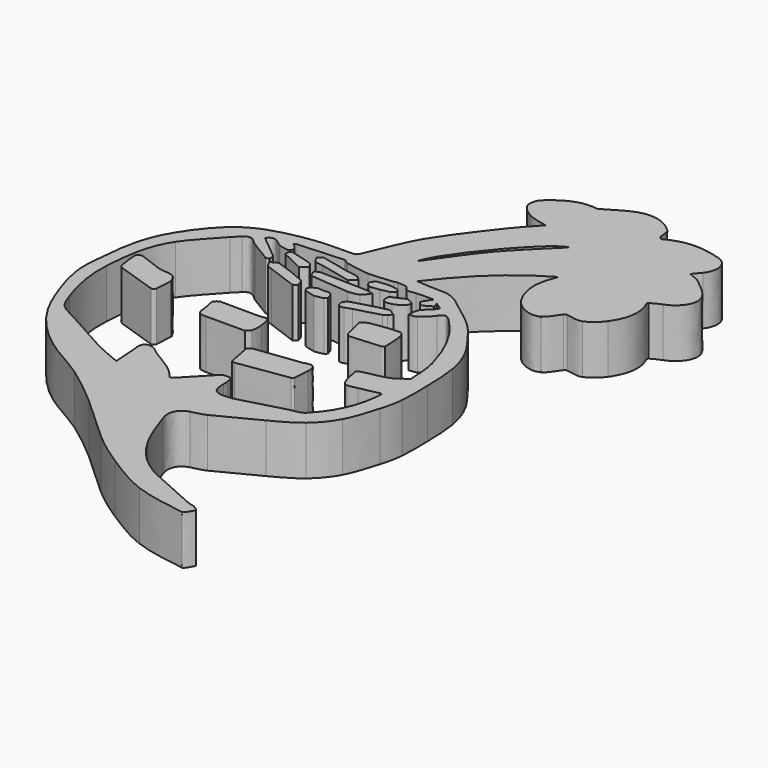
from build123d import *

# Parameters (mm, degrees)
F1_DEPTH = 6.35


# Not quite as in the source:
# - the dataset's text gives a spline's control points without its knots; the knots are read off the source's solid


with BuildPart() as f1:
    # F0 (on Top) → F1 (new body)
    with BuildSketch(Plane.XY):
        with BuildLine():
            add(Edge.make_bspline(
                [(4.2072051852, 31.8483006501), (3.3828085836, 32.0647178316), (2.4756531936, 32.1572918229), (1.7198021082, 32.5450191599)],
                knots=[0, 0, 0, 0, 1, 1, 1, 1], degree=3))
            add(Edge.make_bspline(
                [(1.435188038, 28.715078668), (2.2810654528, 29.8213807729), (3.2804193892, 30.8100077115), (4.2072051852, 31.8483006501)],
                knots=[65, 65, 65, 65, 66, 66, 66, 66], degree=3))
            add(Edge.make_bspline(
                [(-3.5365341043, 21.8426665957), (-2.081577752, 24.2562142926), (-0.2830892938, 26.4680944301), (1.435188038, 28.715078668)],
                knots=[64, 64, 64, 64, 65, 65, 65, 65], degree=3))
            add(Edge.make_bspline(
                [(-6.4304099471, 15.4801891832), (-5.4692441229, 17.6051270032), (-4.731038949, 19.8608537444), (-3.5365341043, 21.8426665957)],
                knots=[63, 63, 63, 63, 64, 64, 64, 64], degree=3))
            add(Edge.make_bspline(
                [(-6.9774600195, 14.832734411), (-6.7812364115, 14.8431127814), (-6.5458860788, 15.2246720946), (-6.4304099471, 15.4801891832)],
                knots=[62, 62, 62, 62, 63, 63, 63, 63], degree=3))
            add(Edge.make_bspline(
                [(-11.8025977362, 14.6692549639), (-10.2139829908, 14.8723974855), (-8.5851956385, 14.7481788505), (-6.9774600195, 14.832734411)],
                knots=[61, 61, 61, 61, 62, 62, 62, 62], degree=3))
            add(Edge.make_bspline(
                [(-17.1400568699, 13.4998244767), (-15.4285107292, 14.0925447424), (-13.6058328909, 14.4388122327), (-11.8025977362, 14.6692549639)],
                knots=[60, 60, 60, 60, 61, 61, 61, 61], degree=3))
            add(Edge.make_bspline(
                [(-20.7615986113, 11.3783461135), (-19.7644168919, 12.3189697367), (-18.4447816174, 13.04808378), (-17.1400568699, 13.4998244767)],
                knots=[59, 59, 59, 59, 60, 60, 60, 60], degree=3))
            add(Edge.make_bspline(
                [(-24.1170571712, 7.1628236841), (-23.1797052822, 8.6861646476), (-22.0579563004, 10.1554683595), (-20.7615986113, 11.3783461135)],
                knots=[58, 58, 58, 58, 59, 59, 59, 59], degree=3))
            add(Edge.make_bspline(
                [(-26.6270137612, -2.7980519719), (-26.4535045711, -0.8760957685), (-26.3074564955, 1.0700766324), (-25.8659064468, 2.9391487364), (-25.5188880666, 4.4080770033), (-24.908173262, 5.8770320878), (-24.1170571712, 7.1628236841)],
                knots=[56, 56, 56, 56, 57, 57, 57, 58, 58, 58, 58], degree=3))
            add(Edge.make_bspline(
                [(-26.5517102363, -5.9227191732), (-26.7292152331, -4.9059070478), (-26.7203118249, -3.8317859364), (-26.6270137612, -2.7980519719)],
                knots=[55, 55, 55, 55, 56, 56, 56, 56], degree=3))
            add(Edge.make_bspline(
                [(-25.4965222761, -9.7386877505), (-25.9495502125, -8.5018112643), (-26.3254778518, -7.2178164401), (-26.5517102363, -5.9227191732)],
                knots=[54, 54, 54, 54, 55, 55, 55, 55], degree=3))
            add(Edge.make_bspline(
                [(-23.6601943331, -13.9141716604), (-24.4193171529, -12.606201996), (-24.9740102113, -11.165083471), (-25.4965222761, -9.7386877505)],
                knots=[53, 53, 53, 53, 54, 54, 54, 54], degree=3))
            add(Edge.make_bspline(
                [(-12.9440039416, -22.9917594966), (-14.5380894559, -21.8721827318), (-16.3289349281, -21.0344846528), (-17.9390036691, -19.9351014615), (-20.2652872386, -18.3466744386), (-22.2420047659, -16.3577549513), (-23.6601943331, -13.9141716604)],
                knots=[51, 51, 51, 51, 52, 52, 52, 53, 53, 53, 53], degree=3))
            add(Edge.make_bspline(
                [(-7.8668085931, -27.0197471862), (-9.4963468352, -25.6031934862), (-11.1786082718, -24.2315322721), (-12.9440039416, -22.9917594966)],
                knots=[50, 50, 50, 50, 51, 51, 51, 51], degree=3))
            add(Edge.make_bspline(
                [(-1.9632053308, -32.4090445369), (-3.985190789, -30.6758566781), (-5.85643511, -28.7673360396), (-7.8668085931, -27.0197471862)],
                knots=[49, 49, 49, 49, 50, 50, 50, 50], degree=3))
            add(Edge.make_bspline(
                [(2.4047209204, -35.6275461519), (0.8784836675, -34.6634840383), (-0.5928313565, -33.5835435306), (-1.9632053308, -32.4090445369)],
                knots=[48, 48, 48, 48, 49, 49, 49, 49], degree=3))
            add(Edge.make_bspline(
                [(8.0590019353, -38.7449458122), (6.0608035948, -38.0082156004), (4.2254142641, -36.7776948605), (2.4047209204, -35.6275461519)],
                knots=[47, 47, 47, 47, 48, 48, 48, 48], degree=3))
            add(Edge.make_bspline(
                [(14.710813297, -40.1737014722), (12.4718206725, -39.8001605899), (10.1690292283, -39.5226263382), (8.0590019353, -38.7449458122)],
                knots=[46, 46, 46, 46, 47, 47, 47, 47], degree=3))
            add(Edge.make_bspline(
                [(15.5905075725, -38.994294877), (15.3333277993, -39.4305886967), (14.9437768726, -40.2124527519), (14.710813297, -40.1737014722)],
                knots=[45, 45, 45, 45, 46, 46, 46, 46], degree=3))
            add(Edge.make_bspline(
                [(14.9466999796, -38.4828852549), (15.1994816837, -38.6003726987), (15.6121492907, -38.9575549094), (15.5905075725, -38.994294877)],
                knots=[44, 44, 44, 44, 45, 45, 45, 45], degree=3))
            add(Edge.make_bspline(
                [(13.8996645377, -38.1624430119), (14.2312092235, -38.3090274374), (14.6187756555, -38.3306691555), (14.9466999796, -38.4828852549)],
                knots=[43, 43, 43, 43, 44, 44, 44, 44], degree=3))
            add(Edge.make_bspline(
                [(8.3861753695, -35.7028496767), (10.2532361613, -36.449421909), (12.0588044381, -37.348934313), (13.8996645377, -38.1624430119)],
                knots=[42, 42, 42, 42, 43, 43, 43, 43], degree=3))
            add(Edge.make_bspline(
                [(2.3654332908, -30.2510139286), (3.7134414746, -32.7353061762), (5.6865386401, -34.6234723364), (8.3861753695, -35.7028496767)],
                knots=[41, 41, 41, 41, 42, 42, 42, 42], degree=3))
            add(Edge.make_bspline(
                [(0.3550866253, -25.2783799915), (0.9492282182, -26.9648249572), (1.5179468263, -28.6887607804), (2.3654332908, -30.2510139286)],
                knots=[40, 40, 40, 40, 41, 41, 41, 41], degree=3))
            add(Edge.make_bspline(
                [(1.596495268, -22.5088836887), (0.624602446, -22.7655002946), (-0.2025295401, -23.6959332699), (0.3550866253, -25.2783799915)],
                knots=[39, 39, 39, 39, 40, 40, 40, 40], degree=3))
            add(Edge.make_bspline(
                [(3.4613838428, -21.9541906303), (2.8857731386, -22.2340848215), (2.2241319117, -22.3430174846), (1.596495268, -22.5088836887)],
                knots=[38, 38, 38, 38, 39, 39, 39, 39], degree=3))
            add(Edge.make_bspline(
                [(8.840839173, -19.1889046742), (7.0685514071, -20.1495073309), (5.2742464781, -21.0725118602), (3.4613838428, -21.9541906303)],
                knots=[37, 37, 37, 37, 38, 38, 38, 38], degree=3))
            add(Edge.make_bspline(
                [(12.2843395677, -17.084509055), (11.2667765524, -17.9418375401), (10.0246170198, -18.5470815758), (8.840839173, -19.1889046742)],
                knots=[36, 36, 36, 36, 37, 37, 37, 37], degree=3))
            add(Edge.make_bspline(
                [(14.6887961339, -14.1671679045), (14.1073660334, -15.2632793615), (13.2371383335, -16.2815664491), (12.2843395677, -17.084509055)],
                knots=[35, 35, 35, 35, 36, 36, 36, 36], degree=3))
            add(Edge.make_bspline(
                [(16.1933916687, -9.9809301792), (15.759645511, -11.4004069861), (15.377174403, -12.869710698), (14.6887961339, -14.1671679045)],
                knots=[34, 34, 34, 34, 35, 35, 35, 35], degree=3))
            add(Edge.make_bspline(
                [(16.7831888276, -7.1594347544), (16.7108084096, -8.110597653), (16.4736613048, -9.0641473087), (16.1933916687, -9.9809301792)],
                knots=[33, 33, 33, 33, 34, 34, 34, 34], degree=3))
            add(Edge.make_bspline(
                [(16.8221010122, -3.0203153671), (16.8652235436, -4.3992173047), (16.8874016116, -5.7863253956), (16.7831888276, -7.1594347544)],
                knots=[32, 32, 32, 32, 33, 33, 33, 33], degree=3))
            add(Edge.make_bspline(
                [(16.5180174409, 1.4059925698), (16.7661060835, -0.0449411583), (16.776109009, -1.5417059846), (16.8221010122, -3.0203153671)],
                knots=[31, 31, 31, 31, 32, 32, 32, 32], degree=3))
            add(Edge.make_bspline(
                [(14.2519659643, 6.5812326786), (15.4364678835, 5.0462529224), (16.1955638858, 3.2919596954), (16.5180174409, 1.4059925698)],
                knots=[30, 30, 30, 30, 31, 31, 31, 31], degree=3))
            add(Edge.make_bspline(
                [(11.639244735, 9.8413818627), (12.630607058, 8.8785801714), (13.4002691532, 7.6849871215), (14.2519659643, 6.5812326786)],
                knots=[29, 29, 29, 29, 30, 30, 30, 30], degree=3))
            add(Edge.make_bspline(
                [(7.9755190746, 12.7578112184), (9.1882061806, 11.773367809), (10.5249510167, 10.9234945875), (11.639244735, 9.8413818627)],
                knots=[28, 28, 28, 28, 29, 29, 29, 29], degree=3))
            add(Edge.make_bspline(
                [(4.9070345244, 14.0116095437), (6.1564615981, 14.0687308072), (7.0721717688, 13.4911087909), (7.9755190746, 12.7578112184)],
                knots=[27, 27, 27, 27, 28, 28, 28, 28], degree=3))
            add(Edge.make_bspline(
                [(1.7237979149, 14.1669364724), (2.8944888244, 14.102172223), (3.9047574811, 13.9657784454), (4.9070345244, 14.0116095437)],
                knots=[26, 26, 26, 26, 27, 27, 27, 27], degree=3))
            add(Edge.make_bspline(
                [(12.295415193, 23.8353941672), (8.0251582571, 21.4389023969), (4.7042674477, 18.1172875152), (1.7237979149, 14.1669364724)],
                knots=[25, 25, 25, 25, 26, 26, 26, 26], degree=3))
            add(Edge.make_bspline(
                [(12.1844712178, 23.4725534652), (12.2253947146, 23.5665756013), (12.245588288, 23.6696888681), (12.295415193, 23.8353941672)],
                knots=[24, 24, 24, 24, 25, 25, 25, 25], degree=3))
            add(Edge.make_bspline(
                [(16.3436232735, 15.9432200451), (15.1894787582, 15.3025232815), (13.3297123249, 16.2014725181), (12.5560276055, 17.4558340107), (11.3502594131, 19.4107220974), (11.2895177879, 21.4037982964), (12.1844712178, 23.4725534652)],
                knots=[22, 22, 22, 22, 23, 23, 23, 24, 24, 24, 24], degree=3))
            add(Edge.make_bspline(
                [(17.8382158828, 17.7450070551), (17.3415290652, 17.1346408779), (16.9785274583, 16.2956823767), (16.3436232735, 15.9432200451)],
                knots=[21, 21, 21, 21, 22, 22, 22, 22], degree=3))
            add(Edge.make_bspline(
                [(18.1317333613, 17.8850211944), (18.036075358, 17.8923155529), (17.9013174476, 17.8226437019), (17.8382158828, 17.7450070551)],
                knots=[20, 20, 20, 20, 21, 21, 21, 21], degree=3))
            add(Edge.make_bspline(
                [(20.247767773, 17.7517114287), (19.6576219868, 17.5136525291), (18.8461246, 17.8317348326), (18.1317333613, 17.8850211944)],
                knots=[19, 19, 19, 19, 20, 20, 20, 20], degree=3))
            add(Edge.make_bspline(
                [(22.2395835498, 19.3877931395), (21.7561713921, 18.7008898327), (21.0141581338, 18.0610780465), (20.247767773, 17.7517114287)],
                knots=[18, 18, 18, 18, 19, 19, 19, 19], degree=3))
            add(Edge.make_bspline(
                [(22.9014124991, 24.8316640918), (23.8280105727, 22.8764005602), (23.4049914128, 21.0438807014), (22.2395835498, 19.3877931395)],
                knots=[17, 17, 17, 17, 18, 18, 18, 18], degree=3))
            add(Edge.make_bspline(
                [(22.9697971104, 25.0764541825), (22.9161353037, 25.0477058283), (22.8728518674, 24.8920302721), (22.9014124991, 24.8316640918)],
                knots=[16, 16, 16, 16, 17, 17, 17, 17], degree=3))
            add(Edge.make_bspline(
                [(24.3003202877, 25.7344482302), (23.8387375706, 25.5623871848), (23.4064395575, 25.3092300357), (22.9697971104, 25.0764541825)],
                knots=[15, 15, 15, 15, 16, 16, 16, 16], degree=3))
            add(Edge.make_bspline(
                [(26.3246925029, 29.5018235072), (27.1167472061, 28.0743550869), (26.0740830158, 26.3957140121), (24.3003202877, 25.7344482302)],
                knots=[14, 14, 14, 14, 15, 15, 15, 15], degree=3))
            add(Edge.make_bspline(
                [(23.8916753049, 31.8932199536), (24.7700823407, 31.16539315), (25.7941888246, 30.4581085473), (26.3246925029, 29.5018235072)],
                knots=[13, 13, 13, 13, 14, 14, 14, 14], degree=3))
            add(Edge.make_bspline(
                [(22.2959539235, 32.6752449137), (22.847402065, 32.4144447787), (23.4540942454, 32.2558729331), (23.8916753049, 31.8932199536)],
                knots=[12, 12, 12, 12, 13, 13, 13, 13], degree=3))
            add(Edge.make_bspline(
                [(23.1245608717, 33.6707907659), (22.8737636622, 33.3428932594), (22.5966048555, 33.0349747864), (22.2959539235, 32.6752449137)],
                knots=[11, 11, 11, 11, 12, 12, 12, 12], degree=3))
            add(Edge.make_bspline(
                [(22.3028728371, 37.1837484717), (23.801836698, 36.7126991789), (24.1828328438, 35.0558875448), (23.1245608717, 33.6707907659)],
                knots=[10, 10, 10, 10, 11, 11, 11, 11], degree=3))
            add(Edge.make_bspline(
                [(15.2715134742, 36.8074722049), (17.5575708018, 38.0938269686), (19.9171348821, 37.9334047158), (22.3028728371, 37.1837484717)],
                knots=[9, 9, 9, 9, 10, 10, 10, 10], degree=3))
            add(Edge.make_bspline(
                [(14.8804875854, 37.0862668788), (14.9163157582, 36.9600637492), (15.207848742, 36.7716440321), (15.2715134742, 36.8074722049)],
                knots=[8, 8, 8, 8, 9, 9, 9, 9], degree=3))
            add(Edge.make_bspline(
                [(14.4791101436, 38.7034422559), (14.8155624309, 38.3771537991), (14.7269842463, 37.6278729998), (14.8804875854, 37.0862668788)],
                knots=[7, 7, 7, 7, 8, 8, 8, 8], degree=3))
            add(Edge.make_bspline(
                [(9.5597625684, 39.8475570282), (11.3797050222, 40.5008311968), (13.1036408454, 40.0372639851), (14.4791101436, 38.7034422559)],
                knots=[6, 6, 6, 6, 7, 7, 7, 7], degree=3))
            add(Edge.make_bspline(
                [(6.3718060798, 38.1323637083), (7.4317407365, 38.712882014), (8.4367263468, 39.4445437193), (9.5597625684, 39.8475570282)],
                knots=[5, 5, 5, 5, 6, 6, 6, 6], degree=3))
            add(Edge.make_bspline(
                [(5.9346004652, 37.9446948811), (6.0671861585, 37.9234017903), (6.231228773, 38.0554511338), (6.3718060798, 38.1323637083)],
                knots=[4, 4, 4, 4, 5, 5, 5, 5], degree=3))
            add(Edge.make_bspline(
                [(0.4269038758, 35.8426592015), (1.9507811892, 37.2623237309), (3.6928992737, 38.303137514), (5.9346004652, 37.9446948811)],
                knots=[3, 3, 3, 3, 4, 4, 4, 4], degree=3))
            add(Edge.make_bspline(
                [(0.053175271, 34.1151030165), (-0.1581465865, 34.5437538503), (0.0559106555, 35.4971157835), (0.4269038758, 35.8426592015)],
                knots=[2, 2, 2, 2, 3, 3, 3, 3], degree=3))
            add(Edge.make_bspline(
                [(1.7198021082, 32.5450191599), (1.0545405195, 32.8862181438), (0.3732688866, 33.4660123771), (0.053175271, 34.1151030165)],
                knots=[1, 1, 1, 1, 2, 2, 2, 2], degree=3))
        make_face()
        with BuildLine():
            add(Edge.make_bspline(
                [(5.5383183474, 12.0670730099), (4.8377381184, 12.0670730099), (4.0335350902, 12.1245429009), (3.2422312769, 12.0485421211)],
                knots=[0, 0, 0, 0, 1, 1, 1, 1], degree=3))
            add(Edge.make_bspline(
                [(4.8126637609, 10.8874786922), (4.9176006173, 11.2450363478), (5.2025901325, 11.5498439915), (5.5383183474, 12.0670730099)],
                knots=[62, 62, 62, 62, 63, 63, 63, 63], degree=3))
            add(Edge.make_bspline(
                [(5.2258677178, 10.2816983066), (5.1560081444, 10.2575089265), (4.7662694953, 10.729630919), (4.8126637609, 10.8874786922)],
                knots=[61, 61, 61, 61, 62, 62, 62, 62], degree=3))
            add(Edge.make_bspline(
                [(6.4632805538, 10.92368231), (6.0846443475, 10.6561509838), (5.6630733323, 10.4320908164), (5.2258677178, 10.2816983066)],
                knots=[60, 60, 60, 60, 61, 61, 61, 61], degree=3))
            add(Edge.make_bspline(
                [(6.335977907, 11.5596591945), (6.3858048119, 11.3316032204), (6.5334887547, 10.9733214925), (6.4632805538, 10.92368231)],
                knots=[59, 59, 59, 59, 60, 60, 60, 60], degree=3))
            add(Edge.make_bspline(
                [(7.2324062991, 10.9711492754), (6.9310581122, 11.2088595476), (6.5933185852, 11.400711904), (6.335977907, 11.5596591945)],
                knots=[58, 58, 58, 58, 59, 59, 59, 59], degree=3))
            add(Edge.make_bspline(
                [(6.8857633638, 10.4097250259), (7.0379794632, 10.5768516522), (7.2540480173, 10.9540397138), (7.2324062991, 10.9711492754)],
                knots=[57, 57, 57, 57, 58, 58, 58, 58], degree=3))
            add(Edge.make_bspline(
                [(5.5686757513, 7.9150544078), (5.6385085073, 8.3718904284), (5.5965123107, 8.8909430364), (5.8072978183, 9.2695792427), (6.0535360538, 9.7119069988), (6.5316651651, 10.021246799), (6.8857633638, 10.4097250259)],
                knots=[55, 55, 55, 55, 56, 56, 56, 57, 57, 57, 57], degree=3))
            add(Edge.make_bspline(
                [(6.6004252213, 8.1231045309), (6.3479921445, 7.9325125967), (5.918214976, 7.9768687328), (5.5686757513, 7.9150544078)],
                knots=[54, 54, 54, 54, 55, 55, 55, 55], degree=3))
            add(Edge.make_bspline(
                [(8.0148067042, 9.5296553054), (7.6519660022, 8.98477745), (7.12856896, 8.5217465882), (6.6004252213, 8.1231045309)],
                knots=[53, 53, 53, 53, 54, 54, 54, 54], degree=3))
            add(Edge.make_bspline(
                [(9.4608328308, 9.5567677925), (8.917778565, 10.0792798573), (8.5491184667, 10.3324370064), (8.0148067042, 9.5296553054)],
                knots=[52, 52, 52, 52, 53, 53, 53, 53], degree=3))
            add(Edge.make_bspline(
                [(14.1312067861, 1.1084524672), (13.2451299469, 4.2718709482), (11.8914900892, 7.218121358), (9.4608328308, 9.5567677925)],
                knots=[51, 51, 51, 51, 52, 52, 52, 52], degree=3))
            add(Edge.make_bspline(
                [(14.5825988553, -2.9208224622), (14.4876649244, -1.5713661337), (14.4912852862, -0.1780632015), (14.1312067861, 1.1084524672)],
                knots=[50, 50, 50, 50, 51, 51, 51, 51], degree=3))
            add(Edge.make_bspline(
                [(13.9344200107, -3.4142375454), (14.1431942062, -3.2287141177), (14.5931381307, -3.0683186825), (14.5825988553, -2.9208224622)],
                knots=[49, 49, 49, 49, 50, 50, 50, 50], degree=3))
            add(Edge.make_bspline(
                [(9.4921020295, -4.9293723556), (10.9808752424, -4.4490442097), (12.6635121239, -4.5447290304), (13.9344200107, -3.4142375454)],
                knots=[48, 48, 48, 48, 49, 49, 49, 49], degree=3))
            add(Edge.make_bspline(
                [(9.2082120316, -5.2334559269), (9.1916656374, -5.1514212109), (9.3717182962, -4.9680968178), (9.4921020295, -4.9293723556)],
                knots=[47, 47, 47, 47, 48, 48, 48, 48], degree=3))
            add(Edge.make_bspline(
                [(9.7600088006, -7.5037177501), (9.4577488189, -6.796245425), (9.362975793, -5.9978349756), (9.2082120316, -5.2334559269)],
                knots=[46, 46, 46, 46, 47, 47, 47, 47], degree=3))
            add(Edge.make_bspline(
                [(11.676708775, -7.8474375785), (11.0223350891, -7.9307327167), (10.1673933611, -8.4574283107), (9.7600088006, -7.5037177501)],
                knots=[45, 45, 45, 45, 46, 46, 46, 46], degree=3))
            add(Edge.make_bspline(
                [(14.1331912807, -7.3189183948), (13.3131659307, -7.4917035125), (12.5043771109, -7.7423129996), (11.676708775, -7.8474375785)],
                knots=[44, 44, 44, 44, 45, 45, 45, 45], degree=3))
            add(Edge.make_bspline(
                [(14.355615581, -7.4586107242), (14.3574391706, -7.4120555536), (14.1979287127, -7.3052951075), (14.1331912807, -7.3189183948)],
                knots=[43, 43, 43, 43, 44, 44, 44, 44], degree=3))
            add(Edge.make_bspline(
                [(10.9636047759, -15.3412914533), (13.0923774976, -13.1767173763), (14.2453956782, -10.5236358175), (14.355615581, -7.4586107242)],
                knots=[42, 42, 42, 42, 43, 43, 43, 43], degree=3))
            add(Edge.make_bspline(
                [(3.4330109335, -17.4738722592), (5.2478580634, -16.9988539773), (7.0550890248, -16.4950605236), (8.863392686, -15.9954774167), (9.5783202746, -15.7979665689), (10.5102013946, -15.8023378205), (10.9636047759, -15.3412914533)],
                knots=[40, 40, 40, 40, 41, 41, 41, 42, 42, 42, 42], degree=3))
            add(Edge.make_bspline(
                [(2.1304584031, -17.6312105001), (2.5669399453, -17.6064579525), (3.0136121354, -17.5835558121), (3.4330109335, -17.4738722592)],
                knots=[39, 39, 39, 39, 40, 40, 40, 40], degree=3))
            add(Edge.make_bspline(
                [(0.5000351836, -15.708127962), (0.4663792279, -17.1226971674), (0.9417729547, -17.698495594), (2.1304584031, -17.6312105001)],
                knots=[38, 38, 38, 38, 39, 39, 39, 39], degree=3))
            add(Edge.make_bspline(
                [(0.4387303909, -14.8460795979), (0.4892813683, -15.1283337286), (0.5067395572, -15.4209662297), (0.5000351836, -15.708127962)],
                knots=[37, 37, 37, 37, 38, 38, 38, 38], degree=3))
            add(Edge.make_bspline(
                [(0.2050427429, -14.149521993), (0.3143240335, -14.1640570751), (0.3943474374, -14.5965428106), (0.4387303909, -14.8460795979)],
                knots=[36, 36, 36, 36, 37, 37, 37, 37], degree=3))
            add(Edge.make_bspline(
                [(-0.9692953458, -14.2528229823), (-0.742124349, -14.0342067662), (-0.1843472787, -14.0974960535), (0.2050427429, -14.149521993)],
                knots=[35, 35, 35, 35, 36, 36, 36, 36], degree=3))
            add(Edge.make_bspline(
                [(-4.3714967988, -17.7810666599), (-3.2357222673, -16.6058167764), (-2.1459665565, -15.3844139846), (-0.9692953458, -14.2528229823)],
                knots=[34, 34, 34, 34, 35, 35, 35, 35], degree=3))
            add(Edge.make_bspline(
                [(-8.9185370965, -14.6562117361), (-7.424856282, -15.5611680915), (-5.8400764383, -16.3421203519), (-4.7881602125, -17.8272463856), (-4.7466735483, -17.8858157938), (-4.4500452405, -17.8621627636), (-4.3714967988, -17.7810666599)],
                knots=[32, 32, 32, 32, 33, 33, 33, 34, 34, 34, 34], degree=3))
            add(Edge.make_bspline(
                [(-9.62027383, -14.1295362552), (-9.3890299262, -14.3072893138), (-9.1614231451, -14.5088898295), (-8.9185370965, -14.6562117361)],
                knots=[31.5, 31.5, 31.5, 31.5, 32, 32, 32, 32], degree=3))
            add(Edge.make_bspline(
                [(-10.3438332997, -13.7459455167), (-10.0863987603, -13.797877595), (-9.8515177338, -13.9517831966), (-9.62027383, -14.1295362552)],
                knots=[31, 31, 31, 31, 31.5, 31.5, 31.5, 31.5], degree=3))
            add(Edge.make_bspline(
                [(-11.3943013809, -14.9184600158), (-11.5316337707, -14.0594956637), (-11.2055330363, -13.5722754217), (-10.3438332997, -13.7459455167)],
                knots=[30, 30, 30, 30, 31, 31, 31, 31], degree=3))
            add(Edge.make_bspline(
                [(-11.2735422027, -16.6764004222), (-11.314277977, -16.0900627201), (-11.301915112, -15.4960820321), (-11.3943013809, -14.9184600158)],
                knots=[29, 29, 29, 29, 30, 30, 30, 30], degree=3))
            add(Edge.make_bspline(
                [(-11.135137113, -18.4830682162), (-11.1840790407, -17.8476276815), (-11.2328064284, -17.2621749568), (-11.2735422027, -16.6764004222)],
                knots=[28, 28, 28, 28, 29, 29, 29, 29], degree=3))
            add(Edge.make_bspline(
                [(-14.6100944289, -16.9764613693), (-13.5094239978, -17.5468158445), (-12.3327527871, -17.9702104494), (-11.135137113, -18.4830682162)],
                knots=[27, 27, 27, 27, 28, 28, 28, 28], degree=3))
            add(Edge.make_bspline(
                [(-19.7947742958, -14.0947874866), (-18.0683176281, -15.0590373226), (-16.3647631009, -16.0671337622), (-14.6100944289, -16.9764613693)],
                knots=[26, 26, 26, 26, 27, 27, 27, 27], degree=3))
            add(Edge.make_bspline(
                [(-22.6508374712, -12.442508009), (-21.8327966157, -13.1485321894), (-20.7583268769, -13.5566408223), (-19.7947742958, -14.0947874866)],
                knots=[25, 25, 25, 25, 26, 26, 26, 26], degree=3))
            add(Edge.make_bspline(
                [(-23.715116562, -10.3684966113), (-23.4519564875, -11.1028668835), (-23.1978875436, -11.9705737389), (-22.6508374712, -12.442508009)],
                knots=[24, 24, 24, 24, 25, 25, 25, 25], degree=3))
            add(Edge.make_bspline(
                [(-24.9385574834, -2.8184332678), (-25.1053354823, -5.4042297325), (-24.5886428138, -7.931832234), (-23.715116562, -10.3684966113)],
                knots=[23, 23, 23, 23, 24, 24, 24, 24], degree=3))
            add(Edge.make_bspline(
                [(-22.7659649755, 5.6457043793), (-24.4749634542, 3.1228217569), (-24.7488505266, 0.1249208526), (-24.9385574834, -2.8184332678)],
                knots=[22, 22, 22, 22, 23, 23, 23, 23], degree=3))
            add(Edge.make_bspline(
                [(-19.1115181682, 9.9034107277), (-20.3465710648, 8.4968331357), (-21.7236762302, 7.1843044973), (-22.7659649755, 5.6457043793)],
                knots=[21, 21, 21, 21, 22, 22, 22, 22], degree=3))
            add(Edge.make_bspline(
                [(-18.2461712523, 10.7725389104), (-18.5469830893, 10.4959164535), (-18.8421632524, 10.210041961), (-19.1115181682, 9.9034107277)],
                knots=[20, 20, 20, 20, 21, 21, 21, 21], degree=3))
            add(Edge.make_bspline(
                [(-16.152878076, 10.2425983995), (-16.7970611139, 10.6510556598), (-17.2831818386, 11.6584280271), (-18.2461712523, 10.7725389104)],
                knots=[19, 19, 19, 19, 20, 20, 20, 20], degree=3))
            add(Edge.make_bspline(
                [(-13.5188905734, 8.6308669737), (-14.4078637021, 9.1495709544), (-15.2835621709, 9.6915257029), (-16.152878076, 10.2425983995)],
                knots=[18, 18, 18, 18, 19, 19, 19, 19], degree=3))
            add(Edge.make_bspline(
                [(-13.0773137073, 8.72381641), (-13.093672379, 8.6563435936), (-13.4163136566, 8.5708494208), (-13.5188905734, 8.6308669737)],
                knots=[17, 17, 17, 17, 18, 18, 18, 18], degree=3))
            add(Edge.make_bspline(
                [(-13.098606798, 9.372719327), (-12.9823797764, 9.2721269047), (-13.026387285, 8.932778328), (-13.0773137073, 8.72381641)],
                knots=[16, 16, 16, 16, 17, 17, 17, 17], degree=3))
            add(Edge.make_bspline(
                [(-16.0937723179, 11.8392047583), (-15.0896716849, 11.0235238424), (-14.0761312938, 10.2189453692), (-13.098606798, 9.372719327)],
                knots=[15, 15, 15, 15, 16, 16, 16, 16], degree=3))
            add(Edge.make_bspline(
                [(-16.2492601516, 11.9370349786), (-16.2239980717, 11.9214003792), (-16.1530657984, 11.8873957961), (-16.0937723179, 11.8392047583)],
                knots=[14, 14, 14, 14, 15, 15, 15, 15], degree=3))
            add(Edge.make_bspline(
                [(-14.196890472, 11.7222536643), (-14.8597921211, 12.0709079116), (-15.3953911234, 13.0097079453), (-16.2492601516, 11.9370349786)],
                knots=[13, 13, 13, 13, 14, 14, 14, 14], degree=3))
            add(Edge.make_bspline(
                [(-12.8658041273, 11.3650714536), (-13.3192075086, 11.4127261416), (-13.7973366199, 11.5120313241), (-14.196890472, 11.7222536643)],
                knots=[12, 12, 12, 12, 13, 13, 13, 13], degree=3))
            add(Edge.make_bspline(
                [(-12.4109526013, 11.8188234624), (-12.4031218929, 11.666607363), (-12.720855569, 11.3497854817), (-12.8658041273, 11.3650714536)],
                knots=[11, 11, 11, 11, 12, 12, 12, 12], degree=3))
            add(Edge.make_bspline(
                [(-12.8041507072, 12.4569993815), (-12.6415562374, 12.2620361957), (-12.4224036715, 12.0394509905), (-12.4109526013, 11.8188234624)],
                knots=[10, 10, 10, 10, 11, 11, 11, 11], degree=3))
            add(Edge.make_bspline(
                [(-13.2319165637, 12.7194353837), (-13.0445695463, 12.6084914085), (-12.8907175798, 12.5608635381), (-12.8041507072, 12.4569993815)],
                knots=[9, 9, 9, 9, 10, 10, 10, 10], degree=3))
            add(Edge.make_bspline(
                [(-12.8518053951, 12.8951167908), (-12.9612744081, 12.8878492498), (-13.0654871921, 12.7989224377), (-13.2319165637, 12.7194353837)],
                knots=[8, 8, 8, 8, 9, 9, 9, 9], degree=3))
            add(Edge.make_bspline(
                [(-6.9594654806, 13.2393997866), (-8.9249196602, 13.1555682984), (-10.8883625277, 13.0226071602), (-12.8518053951, 12.8951167908)],
                knots=[7, 7, 7, 7, 8, 8, 8, 8], degree=3))
            add(Edge.make_bspline(
                [(-6.2496332159, 12.8491247876), (-6.5035144374, 12.8983885252), (-6.7299613618, 13.2492149896), (-6.9594654806, 13.2393997866)],
                knots=[6, 6, 6, 6, 7, 7, 7, 7], degree=3))
            add(Edge.make_bspline(
                [(-3.227355209, 12.3798990845), (-4.2396351778, 12.4142791126), (-5.2482679674, 12.6545102292), (-6.2496332159, 12.8491247876)],
                knots=[5, 5, 5, 5, 6, 6, 6, 6], degree=3))
            add(Edge.make_bspline(
                [(-0.0650362452, 12.6161343944), (-1.1191515056, 12.5250353653), (-2.1768871278, 12.3440709117), (-3.227355209, 12.3798990845)],
                knots=[4, 4, 4, 4, 5, 5, 5, 5], degree=3))
            add(Edge.make_bspline(
                [(0.3621664438, 12.6912501968), (0.2237613542, 12.7054366515), (0.0790005183, 12.6284972595), (-0.0650362452, 12.6161343944)],
                knots=[3, 3, 3, 3, 4, 4, 4, 4], degree=3))
            add(Edge.make_bspline(
                [(1.6903564991, 12.4802769668), (1.5708577432, 12.7163513718), (0.823749161, 12.6446950262), (0.3621664438, 12.6912501968)],
                knots=[2, 2, 2, 2, 3, 3, 3, 3], degree=3))
            add(Edge.make_bspline(
                [(3.2422312769, 12.0485421211), (2.6460515543, 11.9910722302), (2.106108118, 11.6580525822), (1.6903564991, 12.4802769668)],
                knots=[1, 1, 1, 1, 2, 2, 2, 2], degree=3))
        make_face(mode=Mode.SUBTRACT)
        with BuildLine():
            add(Edge.make_bspline(
                [(-1.0005645445, 17.6224242872), (0.4523804957, 19.6360426871), (1.8591189927, 21.8499341367), (3.5361242003, 23.8353941672)],
                knots=[0, 0, 0, 0, 1, 1, 1, 1], degree=3))
            add(Edge.make_bspline(
                [(9.084181119, 29.5412988593), (7.1738368909, 29.4618386227), (-0.585536998, 20.0830903222), (-1.0005645445, 17.6224242872)],
                knots=[2, 2, 2, 2, 3, 3, 3, 3], degree=3))
            add(Edge.make_bspline(
                [(6.2281715786, 26.7104407766), (7.1661536787, 27.644966772), (8.1314628057, 28.572128013), (9.084181119, 29.5412988593)],
                knots=[1.5, 1.5, 1.5, 1.5, 2, 2, 2, 2], degree=3))
            add(Edge.make_bspline(
                [(3.5361242003, 23.8353941672), (4.3795344056, 24.8340240313), (5.2901894786, 25.7759147812), (6.2281715786, 26.7104407766)],
                knots=[1, 1, 1, 1, 1.5, 1.5, 1.5, 1.5], degree=3))
        make_face(mode=Mode.SUBTRACT)
    extrude(amount=F1_DEPTH)


with BuildPart() as f1b:
    # F0 (on Top) → F1, piece 2 (new body)
    with BuildSketch(Plane.XY):
        with BuildLine():
            add(Edge.make_bspline(
                [(5.3858877081, -8.1242477578), (5.33898391, -8.7702275678), (5.3018684975, -9.4171459902), (5.2342347761, -10.0609535831)],
                knots=[0, 0, 0, 0, 1, 1, 1, 1], degree=3))
            add(Edge.make_bspline(
                [(3.9755288494, -6.9693791701), (5.001244383, -6.5885439292), (5.4295465893, -6.9500973915), (5.3858877081, -8.1242477578)],
                knots=[8, 8, 8, 8, 9, 9, 9, 9], degree=3))
            add(Edge.make_bspline(
                [(3.8074636107, -7.0164975081), (3.8645848742, -7.0093908721), (3.9209552478, -6.9895727436), (3.9755288494, -6.9693791701)],
                knots=[7, 7, 7, 7, 8, 8, 8, 8], degree=3))
            add(Edge.make_bspline(
                [(-1.92992482, -7.7303255795), (-0.0210287366, -7.4662537102), (1.8942230931, -7.2494610838), (3.8074636107, -7.0164975081)],
                knots=[6, 6, 6, 6, 7, 7, 7, 7], degree=3))
            add(Edge.make_bspline(
                [(-2.5573469238, -8.2057193064), (-2.5749928352, -8.0707736735), (-2.1674205522, -7.7632306454), (-1.92992482, -7.7303255795)],
                knots=[5, 5, 5, 5, 6, 6, 6, 6], degree=3))
            add(Edge.make_bspline(
                [(-2.3135390238, -9.6789383725), (-2.4086305075, -9.189807384), (-2.4928776668, -8.6989466671), (-2.5573469238, -8.2057193064)],
                knots=[4.5, 4.5, 4.5, 4.5, 5, 5, 5, 5], degree=3))
            add(Edge.make_bspline(
                [(-2.0046651775, -11.1417790682), (-2.112511732, -10.655470621), (-2.2184475401, -10.168069361), (-2.3135390238, -9.6789383725)],
                knots=[4, 4, 4, 4, 4.5, 4.5, 4.5, 4.5], degree=3))
            add(Edge.make_bspline(
                [(-1.5889135586, -11.3072966449), (-1.7225719517, -11.3267393285), (-1.9857588438, -11.2270855185), (-2.0046651775, -11.1417790682)],
                knots=[3, 3, 3, 3, 4, 4, 4, 4], degree=3))
            add(Edge.make_bspline(
                [(4.9819626044, -10.3177579115), (2.7935477747, -10.6600295951), (0.6034970778, -10.991198836), (-1.5889135586, -11.3072966449)],
                knots=[2, 2, 2, 2, 3, 3, 3, 3], degree=3))
            add(Edge.make_bspline(
                [(5.2342347761, -10.0609535831), (5.2240441282, -10.1573356587), (5.0805437145, -10.3022842171), (4.9819626044, -10.3177579115)],
                knots=[1, 1, 1, 1, 2, 2, 2, 2], degree=3))
        make_face()
    extrude(amount=F1_DEPTH)


with BuildPart() as f1c:
    # F0 (on Top) → F1, piece 3 (new body)
    with BuildSketch(Plane.XY):
        with BuildLine():
            add(Edge.make_bspline(
                [(-5.1347763302, -5.1834412994), (-6.9671084666, -5.1834412994), (-8.5497160932, -5.1614241364), (-10.13125102, -5.1934442249)],
                knots=[0, 0, 0, 0, 1, 1, 1, 1], degree=3))
            add(Edge.make_bspline(
                [(-4.6351932232, -4.6409233836), (-4.6964980159, -4.8888243037), (-5.0240200775, -5.0706737346), (-5.1347763302, -5.1834412994)],
                knots=[9, 9, 9, 9, 10, 10, 10, 10], degree=3))
            add(Edge.make_bspline(
                [(-4.5644486725, -3.2263541782), (-4.5146217675, -3.6932199418), (-4.5233374532, -4.1895313144), (-4.6351932232, -4.6409233836)],
                knots=[8, 8, 8, 8, 9, 9, 9, 9], degree=3))
            add(Edge.make_bspline(
                [(-4.954375044, -1.6875663378), (-4.725943625, -2.1542443789), (-4.6208190461, -2.6996585842), (-4.5644486725, -3.2263541782)],
                knots=[7, 7, 7, 7, 8, 8, 8, 8], degree=3))
            add(Edge.make_bspline(
                [(-5.9961006219, -1.7792285343), (-5.6336621824, -1.7416035894), (-5.009297273, -1.5751742179), (-4.954375044, -1.6875663378)],
                knots=[6, 6, 6, 6, 7, 7, 7, 7], degree=3))
            add(Edge.make_bspline(
                [(-6.0841424567, -1.7812398464), (-6.0546700302, -1.7814275689), (-6.0252244211, -1.7821516412), (-5.9961006219, -1.7792285343)],
                knots=[5, 5, 5, 5, 6, 6, 6, 6], degree=3))
            add(Edge.make_bspline(
                [(-11.0093094283, -1.7541541769), (-9.3682932985, -1.7206859436), (-7.7260435639, -1.7632453076), (-6.0841424567, -1.7812398464)],
                knots=[4, 4, 4, 4, 5, 5, 5, 5], degree=3))
            add(Edge.make_bspline(
                [(-11.679290896, -2.3241063897), (-11.6883820267, -2.1364375625), (-11.2490041951, -1.7588740559), (-11.0093094283, -1.7541541769)],
                knots=[3, 3, 3, 3, 4, 4, 4, 4], degree=3))
            add(Edge.make_bspline(
                [(-11.3484702826, -4.2160806341), (-11.3683152286, -3.5828123165), (-11.6483703248, -2.958822852), (-11.679290896, -2.3241063897)],
                knots=[2, 2, 2, 2, 3, 3, 3, 3], degree=3))
            add(Edge.make_bspline(
                [(-10.13125102, -5.1934442249), (-10.8512471151, -5.207979307), (-11.3210091681, -5.0994220888), (-11.3484702826, -4.2160806341)],
                knots=[1, 1, 1, 1, 2, 2, 2, 2], degree=3))
        make_face()
    extrude(amount=F1_DEPTH)


with BuildPart() as f1d:
    # F0 (on Top) → F1, piece 4 (new body)
    with BuildSketch(Plane.XY):
        with BuildLine():
            add(Edge.make_bspline(
                [(-17.7436918559, -1.2527206628), (-17.7900593041, -2.2249889297), (-17.7980509175, -2.8911891306), (-17.8728180924, -3.5500949731)],
                knots=[0, 0, 0, 0, 1, 1, 1, 1], degree=3))
            add(Edge.make_bspline(
                [(-18.4787862005, -0.3004850643), (-18.1019467663, -0.4572333203), (-17.9002792069, -1.0353916865), (-17.7436918559, -1.2527206628)],
                knots=[8, 8, 8, 8, 9, 9, 9, 9], degree=3))
            add(Edge.make_bspline(
                [(-20.5157090032, 0.0638037824), (-19.860611245, -0.1393387393), (-19.100228003, -0.0420448688), (-18.4787862005, -0.3004850643)],
                knots=[7, 7, 7, 7, 8, 8, 8, 8], degree=3))
            add(Edge.make_bspline(
                [(-23.4845129259, 1.1744771389), (-22.482423605, 0.8411088635), (-21.5230813705, 0.3760666895), (-20.5157090032, 0.0638037824)],
                knots=[6, 6, 6, 6, 7, 7, 7, 7], degree=3))
            add(Edge.make_bspline(
                [(-24.0981508375, 0.7803672382), (-24.1021466442, 0.9144010762), (-23.6387403374, 1.2257521886), (-23.4845129259, 1.1744771389)],
                knots=[5, 5, 5, 5, 6, 6, 6, 6], degree=3))
            add(Edge.make_bspline(
                [(-24.0121035538, -0.3771294639), (-24.055276368, 0.0081574811), (-24.0865120448, 0.3942623596), (-24.0981508375, 0.7803672382)],
                knots=[4.5, 4.5, 4.5, 4.5, 5, 5, 5, 5], degree=3))
            add(Edge.make_bspline(
                [(-23.8544334465, -1.5297185645), (-23.9138207883, -1.1468854203), (-23.9689307397, -0.7624164089), (-24.0121035538, -0.3771294639)],
                knots=[4, 4, 4, 4, 4.5, 4.5, 4.5, 4.5], degree=3))
            add(Edge.make_bspline(
                [(-23.5236128331, -2.1493367774), (-23.6900153871, -2.0904187417), (-23.819704791, -1.7543150818), (-23.8544334465, -1.5297185645)],
                knots=[3, 3, 3, 3, 4, 4, 4, 4], degree=3))
            add(Edge.make_bspline(
                [(-18.297285397, -3.8914548619), (-20.0483068898, -3.3383976706), (-21.7929726362, -2.7631355939), (-23.5236128331, -2.1493367774)],
                knots=[2, 2, 2, 2, 3, 3, 3, 3], degree=3))
            add(Edge.make_bspline(
                [(-17.8728180924, -3.5500949731), (-17.8880772469, -3.6850406059), (-18.1950839251, -3.9238235779), (-18.297285397, -3.8914548619)],
                knots=[1, 1, 1, 1, 2, 2, 2, 2], degree=3))
        make_face()
    extrude(amount=F1_DEPTH)


with BuildPart() as f1e:
    # F0 (on Top) → F1, piece 5 (new body)
    with BuildSketch(Plane.XY):
        with BuildLine():
            add(Edge.make_bspline(
                [(-7.6794883933, 5.687164226), (-8.9710993859, 6.1587498686), (-10.2458153569, 6.6214052855), (-11.517983666, 7.0911673385)],
                knots=[0, 0, 0, 0, 1, 1, 1, 1], degree=3))
            add(Edge.make_bspline(
                [(-7.1662551815, 6.0119777206), (-7.1531682441, 5.9770613427), (-7.462159417, 5.8221098588), (-7.6794883933, 5.687164226)],
                knots=[6, 6, 6, 6, 7, 7, 7, 7], degree=3))
            add(Edge.make_bspline(
                [(-7.6665623609, 7.0082476452), (-7.3981192399, 6.8871130221), (-7.2981168025, 6.3658881969), (-7.1662551815, 6.0119777206)],
                knots=[5, 5, 5, 5, 6, 6, 6, 6], degree=3))
            add(Edge.make_bspline(
                [(-11.5740054122, 8.5157394694), (-10.2469148742, 8.0847286961), (-8.9380065976, 7.5824102047), (-7.6665623609, 7.0082476452)],
                knots=[4, 4, 4, 4, 5, 5, 5, 5], degree=3))
            add(Edge.make_bspline(
                [(-12.0495499875, 8.4050804301), (-11.8734361482, 8.4961492896), (-11.7065776968, 8.5587547308), (-11.5740054122, 8.5157394694)],
                knots=[3.5, 3.5, 3.5, 3.5, 4, 4, 4, 4], degree=3))
            add(Edge.make_bspline(
                [(-12.5806268897, 8.1236408808), (-12.4110330538, 8.1944792928), (-12.2256638267, 8.3140115706), (-12.0495499875, 8.4050804301)],
                knots=[3, 3, 3, 3, 3.5, 3.5, 3.5, 3.5], degree=3))
            add(Edge.make_bspline(
                [(-12.1941599749, 7.4089010146), (-12.3774843681, 7.5926008526), (-12.4564082547, 7.8808621021), (-12.5806268897, 8.1236408808)],
                knots=[2, 2, 2, 2, 3, 3, 3, 3], degree=3))
            add(Edge.make_bspline(
                [(-11.517983666, 7.0911673385), (-11.7533071811, 7.178109656), (-12.0284814933, 7.242847088), (-12.1941599749, 7.4089010146)],
                knots=[1, 1, 1, 1, 2, 2, 2, 2], degree=3))
        make_face()
    extrude(amount=F1_DEPTH)


with BuildPart() as f1f:
    # F0 (on Top) → F1, piece 6 (new body)
    with BuildSketch(Plane.XY):
        with BuildLine():
            add(Edge.make_bspline(
                [(-9.5494454745, 9.1233702622), (-10.5438918095, 9.5871251964), (-11.4781596865, 10.0014286705), (-12.3818556197, 10.4739261079)],
                knots=[0, 0, 0, 0, 1, 1, 1, 1], degree=3))
            add(Edge.make_bspline(
                [(-8.6988481807, 9.7868350787), (-8.9561888589, 9.5860524966), (-9.2137172596, 9.3852699145), (-9.5494454745, 9.1233702622)],
                knots=[5, 5, 5, 5, 6, 6, 6, 6], degree=3))
            add(Edge.make_bspline(
                [(-11.960472327, 11.2328612052), (-11.0818507512, 11.0107855324), (-10.1961761744, 10.8001877473), (-9.3446670857, 10.4964796209), (-9.0789593492, 10.401706595), (-8.9114572779, 10.031062002), (-8.6988481807, 9.7868350787)],
                knots=[3, 3, 3, 3, 4, 4, 4, 5, 5, 5, 5], degree=3))
            add(Edge.make_bspline(
                [(-12.397865664, 11.1359159623), (-12.3834914869, 11.2006533942), (-12.0968661045, 11.2674021383), (-11.960472327, 11.2328612052)],
                knots=[2, 2, 2, 2, 3, 3, 3, 3], degree=3))
            add(Edge.make_bspline(
                [(-12.3818556197, 10.4739261079), (-12.4829843918, 10.5266493023), (-12.4460567018, 10.9182115411), (-12.397865664, 11.1359159623)],
                knots=[1, 1, 1, 1, 2, 2, 2, 2], degree=3))
        make_face()
    extrude(amount=F1_DEPTH)


with BuildPart() as f1g:
    # F0 (on Top) → F1, piece 7 (new body)
    with BuildSketch(Plane.XY):
        with BuildLine():
            add(Edge.make_bspline(
                [(-3.9324675946, 9.9828709642), (-5.3346471175, 10.3022405075), (-6.6221013985, 10.6001292375), (-7.912076524, 10.8860305475)],
                knots=[0, 0, 0, 0, 1, 1, 1, 1], degree=3))
            add(Edge.make_bspline(
                [(-3.1320458332, 10.7059778888), (-3.3953936302, 10.4681067116), (-3.6589291497, 10.230047812), (-3.9324675946, 9.9828709642)],
                knots=[7, 7, 7, 7, 8, 8, 8, 8], degree=3))
            add(Edge.make_bspline(
                [(-3.7811364726, 11.2228582798), (-3.5347105146, 11.1422717085), (-3.3462907976, 10.8842069579), (-3.1320458332, 10.7059778888)],
                knots=[6, 6, 6, 6, 7, 7, 7, 7], degree=3))
            add(Edge.make_bspline(
                [(-5.0423900613, 11.4378273165), (-4.6261020926, 11.3448778802), (-4.1819775644, 11.3539690109), (-3.7811364726, 11.2228582798)],
                knots=[5, 5, 5, 5, 6, 6, 6, 6], degree=3))
            add(Edge.make_bspline(
                [(-8.8107039507, 12.2884246104), (-7.5474390498, 12.0423472799), (-6.2994601209, 11.7182578576), (-5.0423900613, 11.4378273165)],
                knots=[4, 4, 4, 4, 5, 5, 5, 5], degree=3))
            add(Edge.make_bspline(
                [(-9.5034266538, 11.9186918123), (-9.2709994281, 12.0498025434), (-9.0100383881, 12.3271490726), (-8.8107039507, 12.2884246104)],
                knots=[3, 3, 3, 3, 4, 4, 4, 4], degree=3))
            add(Edge.make_bspline(
                [(-8.9800296116, 11.0970037776), (-9.2290032315, 11.2484958046), (-9.3344764378, 11.6356867917), (-9.5034266538, 11.9186918123)],
                knots=[2, 2, 2, 2, 3, 3, 3, 3], degree=3))
            add(Edge.make_bspline(
                [(-7.912076524, 10.8860305475), (-8.2696341795, 10.9653298791), (-8.6892207001, 10.9202228531), (-8.9800296116, 11.0970037776)],
                knots=[1, 1, 1, 1, 2, 2, 2, 2], degree=3))
        make_face()
    extrude(amount=F1_DEPTH)


with BuildPart() as f1h:
    # F0 (on Top) → F1, piece 8 (new body)
    with BuildSketch(Plane.XY):
        with BuildLine():
            add(Edge.make_bspline(
                [(-2.3454887164, 7.9850480687), (-4.1574395569, 8.1292725547), (-5.7409589783, 8.2285777372), (-7.3139391243, 8.415897937)],
                knots=[0, 0, 0, 0, 1, 1, 1, 1], degree=3))
            add(Edge.make_bspline(
                [(-0.9887380294, 8.2558511292), (-1.4517957087, 8.030718262), (-2.0286668351, 8.0399971151), (-2.3454887164, 7.9850480687)],
                knots=[6, 6, 6, 6, 7, 7, 7, 7], degree=3))
            add(Edge.make_bspline(
                [(-0.1363439634, 9.2348505872), (-0.4153263597, 8.8976742276), (-0.6306440239, 8.4300843916), (-0.9887380294, 8.2558511292)],
                knots=[5, 5, 5, 5, 6, 6, 6, 6], degree=3))
            add(Edge.make_bspline(
                [(-1.1911564786, 9.4354454469), (-0.8376214473, 9.4227339544), (-0.4878945001, 9.3043347158), (-0.1363439634, 9.2348505872)],
                knots=[4, 4, 4, 4, 5, 5, 5, 5], degree=3))
            add(Edge.make_bspline(
                [(-4.1499306584, 9.5292128168), (-3.1635228675, 9.502931672), (-2.177249164, 9.4707372698), (-1.1911564786, 9.4354454469)],
                knots=[3.5, 3.5, 3.5, 3.5, 4, 4, 4, 4], degree=3))
            add(Edge.make_bspline(
                [(-7.1095093629, 9.5875006413), (-6.1228803277, 9.5758618486), (-5.1363384493, 9.5554939615), (-4.1499306584, 9.5292128168)],
                knots=[3, 3, 3, 3, 3.5, 3.5, 3.5, 3.5], degree=3))
            add(Edge.make_bspline(
                [(-7.7513056438, 9.2279316736), (-7.7682274829, 9.298327597), (-7.3339449753, 9.5900483033), (-7.1095093629, 9.5875006413)],
                knots=[2, 2, 2, 2, 3, 3, 3, 3], degree=3))
            add(Edge.make_bspline(
                [(-7.3139391243, 8.415897937), (-7.5008838792, 8.4381028225), (-7.6794883933, 8.9282193539), (-7.7513056438, 9.2279316736)],
                knots=[1, 1, 1, 1, 2, 2, 2, 2], degree=3))
        make_face()
    extrude(amount=F1_DEPTH)


with BuildPart() as f1i:
    # F0 (on Top) → F1, piece 9 (new body)
    with BuildSketch(Plane.XY):
        with BuildLine():
            add(Edge.make_bspline(
                [(-4.4222354986, 5.1611927043), (-4.8336158658, 5.2632332713), (-5.3353980074, 5.3436053026), (-5.7958812072, 5.5273051407)],
                knots=[0, 0, 0, 0, 1, 1, 1, 1], degree=3))
            add(Edge.make_bspline(
                [(-3.3261240416, 5.3777976082), (-3.6454667674, 5.2765079311), (-3.9859148614, 5.2415915531), (-4.4222354986, 5.1611927043)],
                knots=[6, 6, 6, 6, 7, 7, 7, 7], degree=3))
            add(Edge.make_bspline(
                [(-3.0651361841, 5.7271759279), (-3.0418585988, 5.6329660694), (-3.2082611528, 5.4150739257), (-3.3261240416, 5.3777976082)],
                knots=[5, 5, 5, 5, 6, 6, 6, 6], degree=3))
            add(Edge.make_bspline(
                [(-4.7139897268, 6.6798607194), (-4.5503493747, 6.6491010531), (-4.3854821222, 6.6165915453), (-4.2385356605, 6.6523258568), (-3.413602709, 6.8529207165), (-3.2115328872, 6.3211566159), (-3.0651361841, 5.7271759279)],
                knots=[3.5, 3.5, 3.5, 3.5, 4, 4, 4, 5, 5, 5, 5], degree=3))
            add(Edge.make_bspline(
                [(-5.1820823907, 6.6968965328), (-5.0400435305, 6.7396302105), (-4.8776300788, 6.7106203857), (-4.7139897268, 6.6798607194)],
                knots=[3, 3, 3, 3, 3.5, 3.5, 3.5, 3.5], degree=3))
            add(Edge.make_bspline(
                [(-6.0695805572, 6.0974450759), (-5.8186224426, 6.3477059356), (-5.5130639091, 6.5972159054), (-5.1820823907, 6.6968965328)],
                knots=[2, 2, 2, 2, 3, 3, 3, 3], degree=3))
            add(Edge.make_bspline(
                [(-5.7958812072, 5.5273051407), (-5.9488213789, 5.5882344884), (-6.1241541587, 6.0430860144), (-6.0695805572, 6.0974450759)],
                knots=[1, 1, 1, 1, 2, 2, 2, 2], degree=3))
        make_face()
    extrude(amount=F1_DEPTH)


with BuildPart() as f1j:
    # F0 (on Top) → F1, piece 10 (new body)
    with BuildSketch(Plane.XY):
        with BuildLine():
            add(Edge.make_bspline(
                [(-1.3670256083, 5.8493832509), (-1.2671840759, 5.9570554917), (-1.1111330747, 6.2798576742), (-0.878705849, 6.350602225)],
                knots=[0, 0, 0, 0, 1, 1, 1, 1], degree=3))
            add(Edge.make_bspline(
                [(-0.4705972161, 5.0527963911), (-1.0533145564, 4.832383403), (-1.3106552346, 5.0771734937), (-1.3670256083, 5.8493832509)],
                knots=[6, 6, 6, 6, 7, 7, 7, 7], degree=3))
            add(Edge.make_bspline(
                [(0.3850685842, 5.3397972184), (0.0951714676, 5.2608733318), (-0.1892548802, 5.1590204873), (-0.4705972161, 5.0527963911)],
                knots=[5, 5, 5, 5, 6, 6, 6, 6], degree=3))
            add(Edge.make_bspline(
                [(3.5926822964, 6.2207519161), (2.5400419982, 5.8764957379), (1.4551938889, 5.6316788297), (0.3850685842, 5.3397972184)],
                knots=[4, 4, 4, 4, 5, 5, 5, 5], degree=3))
            add(Edge.make_bspline(
                [(4.0129593675, 6.526638964), (3.8841281234, 6.3902116645), (3.7493635086, 6.2719465133), (3.5926822964, 6.2207519161)],
                knots=[3.5, 3.5, 3.5, 3.5, 4, 4, 4, 4], degree=3))
            add(Edge.make_bspline(
                [(4.3976362144, 6.9414989011), (4.2646884849, 6.817655711), (4.1417906115, 6.6630662634), (4.0129593675, 6.526638964)],
                knots=[3, 3, 3, 3, 3.5, 3.5, 3.5, 3.5], degree=3))
            add(Edge.make_bspline(
                [(3.3724302132, 7.4982032716), (3.6614423526, 7.5600444142), (4.0533532187, 7.1395460988), (4.3976362144, 6.9414989011)],
                knots=[2, 2, 2, 2, 3, 3, 3, 3], degree=3))
            add(Edge.make_bspline(
                [(-0.878705849, 6.350602225), (0.5260213359, 6.7776440091), (1.9386060467, 7.1919474832), (3.3724302132, 7.4982032716)],
                knots=[1, 1, 1, 1, 2, 2, 2, 2], degree=3))
        make_face()
    extrude(amount=F1_DEPTH)


with BuildPart() as f1k:
    # F0 (on Top) → F1, piece 11 (new body)
    with BuildSketch(Plane.XY):
        with BuildLine():
            add(Edge.make_bspline(
                [(3.0936355393, 2.2916939641), (3.0003374756, 2.7343435301), (2.6942694096, 3.4345483142), (2.8561129896, 3.5682067073), (3.2456907337, 3.8899361901), (3.8440158558, 4.0110708132), (4.3769062911, 4.0958140962)],
                knots=[0, 0, 0, 0, 1, 1, 1, 2, 2, 2, 2], degree=3))
            add(Edge.make_bspline(
                [(3.0630904129, 2.2851504954), (3.0732810609, 2.2873227125), (3.0834448913, 2.2894949296), (3.0936355393, 2.2916939641)],
                knots=[9, 9, 9, 9, 10, 10, 10, 10], degree=3))
            add(Edge.make_bspline(
                [(3.353336157, 1.0984495417), (3.271515981, 1.4971184165), (3.1607597283, 1.889753355), (3.0630904129, 2.2851504954)],
                knots=[8, 8, 8, 8, 9, 9, 9, 9], degree=3))
            add(Edge.make_bspline(
                [(8.107729323, 0.9997075266), (8.1099283576, 0.9205959175), (7.9043990789, 0.7720001799), (7.786911635, 0.7625336043), (6.6386133336, 0.6699864304), (5.4822966012, 0.6496051345), (4.3419899131, 0.5032084315), (3.7738344724, 0.4302648461), (3.4700995285, 0.5283096064), (3.353336157, 1.0984495417)],
                knots=[5, 5, 5, 5, 6, 6, 6, 7, 7, 7, 8, 8, 8, 8], degree=3))
            add(Edge.make_bspline(
                [(7.9444107809, 3.6553367473), (8.0673689936, 2.779289651), (8.0809922809, 1.8866693431), (8.107729323, 0.9997075266)],
                knots=[4, 4, 4, 4, 5, 5, 5, 5], degree=3))
            add(Edge.make_bspline(
                [(7.3464342862, 4.3933541988), (7.548665013, 4.3980740778), (7.9051231513, 3.9364913607), (7.9444107809, 3.6553367473)],
                knots=[3, 3, 3, 3, 4, 4, 4, 4], degree=3))
            add(Edge.make_bspline(
                [(4.3769062911, 4.0958140962), (5.3593383884, 4.2520528197), (6.3541601683, 4.3697011686), (7.3464342862, 4.3933541988)],
                knots=[2, 2, 2, 2, 3, 3, 3, 3], degree=3))
        make_face()
    extrude(amount=F1_DEPTH)


with BuildPart() as f1l:
    # F0 (on Top) → F1, piece 12 (new body)
    with BuildSketch(Plane.XY):
        with BuildLine():
            add(Edge.make_bspline(
                [(0.2819553175, 11.7135379785), (0.6031484504, 11.6556926427), (0.9119519007, 11.639333971), (1.1876625628, 11.5351211869)],
                knots=[0, 0, 0, 0, 1, 1, 1, 1], degree=3))
            add(Edge.make_bspline(
                [(-1.3779403286, 11.537132499), (-0.8408931816, 11.6829660347), (-0.2596508036, 11.6662587356), (0.2819553175, 11.7135379785)],
                knots=[6, 6, 6, 6, 7, 7, 7, 7], degree=3))
            add(Edge.make_bspline(
                [(-1.8964565867, 10.8398508218), (-1.9339206267, 11.0444414882), (-1.6125665889, 11.4734677668), (-1.3779403286, 11.537132499)],
                knots=[5, 5, 5, 5, 6, 6, 6, 6], degree=3))
            add(Edge.make_bspline(
                [(-1.2308195532, 10.2320323066), (-1.4554160705, 10.2189453692), (-1.8513495608, 10.5932371414), (-1.8964565867, 10.8398508218)],
                knots=[4, 4, 4, 4, 5, 5, 5, 5], degree=3))
            add(Edge.make_bspline(
                [(-0.0784751622, 10.374614221), (-0.4610568924, 10.3058675736), (-0.8458007831, 10.2544919583), (-1.2308195532, 10.2320323066)],
                knots=[3.5, 3.5, 3.5, 3.5, 4, 4, 4, 4], degree=3))
            add(Edge.make_bspline(
                [(1.0608962658, 10.6214223283), (0.6845261377, 10.529478548), (0.304106568, 10.4433608685), (-0.0784751622, 10.374614221)],
                knots=[3, 3, 3, 3, 3.5, 3.5, 3.5, 3.5], degree=3))
            add(Edge.make_bspline(
                [(1.6055863987, 11.1344678175), (1.4255605574, 10.9569628208), (1.2716817733, 10.6728851004), (1.0608962658, 10.6214223283)],
                knots=[2, 2, 2, 2, 3, 3, 3, 3], degree=3))
            add(Edge.make_bspline(
                [(1.1876625628, 11.5351211869), (1.3537164893, 11.4723682496), (1.4680931038, 11.2726851847), (1.6055863987, 11.1344678175)],
                knots=[1, 1, 1, 1, 2, 2, 2, 2], degree=3))
        make_face()
    extrude(amount=F1_DEPTH)


with BuildPart() as f1m:
    # F0 (on Top) → F1, piece 13 (new body)
    with BuildSketch(Plane.XY):
        with BuildLine():
            add(Edge.make_bspline(
                [(3.3966195933, 10.5048466792), (3.6383256722, 10.3853479233), (4.0742708645, 10.3102321209), (4.2343176723, 10.0594349113)],
                knots=[0, 0, 0, 0, 1, 1, 1, 1], degree=3))
            add(Edge.make_bspline(
                [(1.7230738425, 9.7566385798), (2.2335984873, 10.0208981716), (2.7713697066, 10.2324077515), (3.3966195933, 10.5048466792)],
                knots=[4, 4, 4, 4, 5, 5, 5, 5], degree=3))
            add(Edge.make_bspline(
                [(1.5712331881, 9.2926959231), (1.5605061902, 9.4483714793), (1.6176006363, 9.7022527007), (1.7230738425, 9.7566385798)],
                knots=[3, 3, 3, 3, 4, 4, 4, 4], degree=3))
            add(Edge.make_bspline(
                [(1.9970648327, 8.6038651089), (1.7670478293, 8.6579258258), (1.602596248, 8.840660234), (1.5712331881, 9.2926959231)],
                knots=[2.5, 2.5, 2.5, 2.5, 3, 3, 3, 3], degree=3))
            add(Edge.make_bspline(
                [(2.8162890101, 8.6870764424), (2.5226642617, 8.6244173663), (2.2270818361, 8.5498043919), (1.9970648327, 8.6038651089)],
                knots=[2, 2, 2, 2, 2.5, 2.5, 2.5, 2.5], degree=3))
            add(Edge.make_bspline(
                [(4.2343176723, 10.0594349113), (4.5153113808, 9.6194939123), (3.7030899217, 8.8760325094), (2.8162890101, 8.6870764424)],
                knots=[1, 1, 1, 1, 2, 2, 2, 2], degree=3))
        make_face()
    extrude(amount=F1_DEPTH)


solid = Compound([f1.part, f1b.part, f1c.part, f1d.part, f1e.part, f1f.part, f1g.part, f1h.part, f1i.part, f1j.part, f1k.part, f1l.part, f1m.part])
